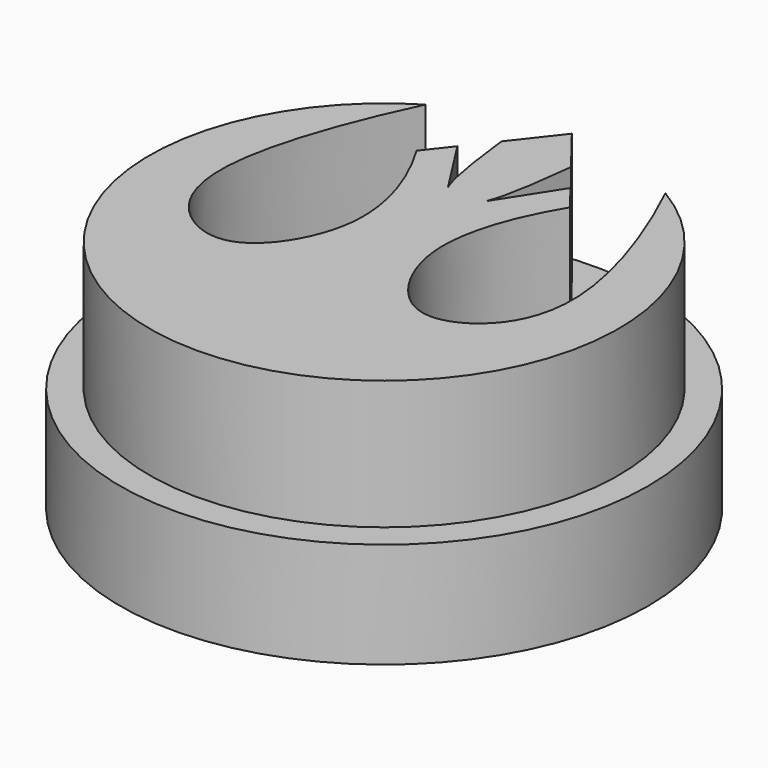
from build123d import *

# Parameters (mm, degrees)
F1_R     = 28.575
F2_DEPTH = 25.4
F0_R     = 28.575
F3_DEPTH = 13.97
F4_SCALE = 0.1777778


with BuildPart() as f2:
    # F1 (on Top) → F2 (new body)
    with BuildSketch(Plane.XY):
        Circle(F1_R)
    extrude(amount=-F2_DEPTH)

    # F0 (on Top) → F3 (cut)
    with BuildSketch(Plane.XY):
        Circle(F0_R)
        with BuildLine():
            ThreePointArc((0, 25.4), (6.7319690535, 24.491643323), (12.9824397575, 21.8315427293))
            ThreePointArc((12.9824397575, 21.8315427293), (22.0784280446, 12.5579861076), (25.4, 0))
            ThreePointArc((25.4, 0), (-12.5579861076, -22.0784280446), (-12.9824397575, 21.8315427293))
            ThreePointArc((-12.9824397575, 21.8315427293), (-6.7319690535, 24.491643323), (0, 25.4))
        make_face(mode=Mode.SUBTRACT)
        with BuildLine():
            Line((-3.7666436157, 20.576738125), (0, 25.4))
            ThreePointArc((0, 25.4), (-6.7319690535, 24.491643323), (-12.9824397575, 21.8315427293))
            add(Edge.make_bspline(
                [(-12.9824397575, 21.8315427293), (-16.0030685137, 15.555784787), (-20.8706185969, 2.5324190308), (-17.0205320702, -6.8009951083), (-9.0413114467, -9.8024376533), (-2.0221816541, 1.6054390369), (-6.0604248598, 11.0668484831), (-8.3033278917, 14.767423908)],
                knots=[0, 0, 0, 0, 0.267130235, 0.4415507763, 0.5882558694, 0.7799558658, 1, 1, 1, 1], degree=3))
            Line((-8.3033278917, 14.767423908), (-6.1221701965, 17.5604396079))
            Line((-6.1221701965, 17.5604396079), (-2.0420027431, 11.1948987469))
            add(Edge.make_bspline(
                [(-3.7666436157, 20.576738125), (-3.3145767707, 16.8504529935), (-2.8625099256, 13.1241678621), (-2.0420027431, 11.1948987469)],
                knots=[0, 0, 0, 0, 0.6621620022, 0.6621620022, 0.6621620022, 0.6621620022], degree=3))
        make_face()
        with BuildLine():
            Line((6.1221701965, 17.5604396079), (8.3033278917, 14.767423908))
            add(Edge.make_bspline(
                [(12.9824397575, 21.8315427293), (16.0030685137, 15.555784787), (20.8706185969, 2.5324190308), (17.0205320702, -6.8009951083), (9.0413114467, -9.8024376533), (2.0221816541, 1.6054390369), (6.0604248598, 11.0668484831), (8.3033278917, 14.767423908)],
                knots=[0, 0, 0, 0, 0.267130235, 0.4415507763, 0.5882558694, 0.7799558658, 1, 1, 1, 1], degree=3))
            ThreePointArc((12.9824397575, 21.8315427293), (6.7319690535, 24.491643323), (0, 25.4))
            Line((0, 25.4), (3.7666436157, 20.576738125))
            add(Edge.make_bspline(
                [(3.7666436157, 20.576738125), (3.3145767707, 16.8504529935), (2.8625099256, 13.1241678621), (2.0420027431, 11.1948987469)],
                knots=[0, 0, 0, 0, 0.6621620022, 0.6621620022, 0.6621620022, 0.6621620022], degree=3))
            Line((2.0420027431, 11.1948987469), (6.1221701965, 17.5604396079))
        make_face()
    extrude(amount=-F3_DEPTH, mode=Mode.SUBTRACT)


with BuildPart() as f2_1:
    # F4: moved
    add(f2.part.scale(F4_SCALE))


solid = f2_1.part
